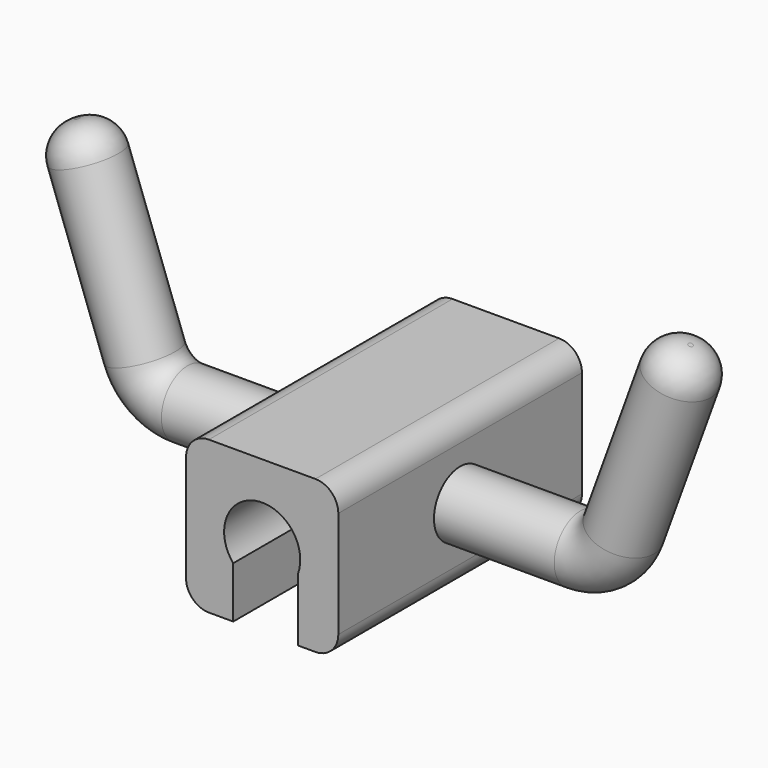
from build123d import *

# Parameters (mm, degrees)
F0_W     = 10
F0_H     = 10
F1_DEPTH = 10
F4_R     = 2.15
F3_R     = 2.5
F7_DEPTH = 25
F8_W     = 4.25
F8_H     = 1.8911467679
F9_DEPTH = 63
F10_R    = 1.5
F11_R    = 2


# Not quite as in the source:
# - an extrude ends at something that could not be found from the text; its depth is read off the source's solid


with BuildPart() as f1:
    # F0 (on Front) → F1 (new body, symmetric)
    with BuildSketch(Plane.XZ):
        Rectangle(F0_W, F0_H)
    extrude(amount=F1_DEPTH, both=True)

    # F5: sweep along a path in F2
    with BuildLine(Plane.XZ) as f5_path:
        Line((0, 0), (12.8993773854, 0))
        ThreePointArc((12.8993773854, 0), (14.6201066944, 0.5425438671), (15.7184552477, 1.97393957))
        Line((15.7184552477, 1.97393957), (20.1303021499, 14.0953893118))
    # F4 (on face) → F5 (sweep)
    with BuildSketch(Plane.YZ.offset(5)):
        Circle(F4_R)
    sweep(path=f5_path.line)

    # F6: F1 across plane


with BuildPart() as f1_1:
    add(f1.part)
    add(f1.part.mirror(Plane.YZ))

    # F3 (on face) → F7 (cut)
    with BuildSketch(Plane.XZ.offset(10)):
        Circle(F3_R)
    extrude(amount=-F7_DEPTH, mode=Mode.SUBTRACT)

    # F8 (on face) → F9 (cut, through all)
    with BuildSketch(Plane.XZ.offset(10)):
        with Locations((0.225, -5.9455733839)):
            Rectangle(F8_W, F8_H)
        with BuildLine():
            Line((-1.9, -1.6248076809), (-1.9, -5))
            Line((-1.9, -5), (2.35, -5))
            Line((2.35, -5), (2.35, -0.8529361055))
            ThreePointArc((2.35, -0.8529361055), (0.4467341852, -2.4597618925), (-1.9, -1.6248076809))
        make_face()
        with BuildLine():
            Line((-1.9, 0), (-1.9, -1.6248076809))
            ThreePointArc((-1.9, -1.6248076809), (0.4467341852, -2.4597618925), (2.35, -0.8529361055))
            Line((2.35, -0.8529361055), (2.35, 0))
            Line((2.35, 0), (-1.9, 0))
        make_face()
    extrude(amount=-F9_DEPTH, mode=Mode.SUBTRACT)

    # F10
    f10_edges = [f1_1.edges().sort_by_distance(p)[0] for p in [
        (5, 0, 5),
        (-5, 0, 5),
        (5, 0, -5),
        (-5, 0, -5),
    ]]
    fillet(f10_edges, radius=F10_R)

    # F11
    f11_edges = [f1_1.edges().sort_by_distance(p)[0] for p in [
        (-20.130302, -2.15, 14.095389),
        (20.130302, -2.15, 14.095389),
    ]]
    fillet(f11_edges, radius=F11_R)


solid = f1_1.part
